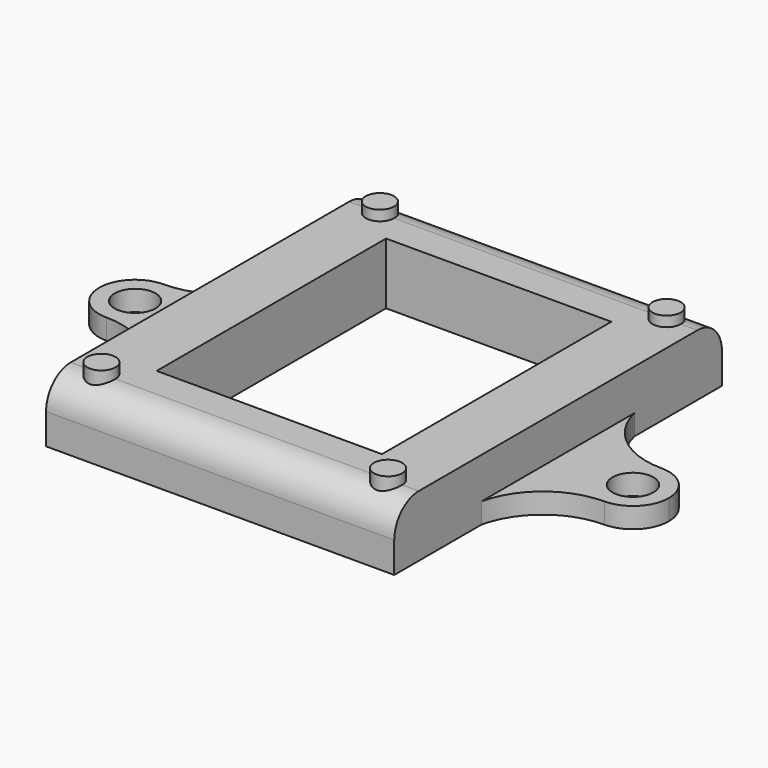
from build123d import *

# Parameters (mm, degrees)
F0_R         = 2.54
F1_DEPTH     = 2.54
F0_R_2       = 1.7526
F0_W         = 27.94
F0_H         = 35.56
F2_DEPTH     = 7.62
F3_DEPTH     = 8.89
F4_T4_DEPTH  = 62.23
F4_S5_R      = 1.7526
F4_T6_DEPTH  = 33
F4_S7_R      = 1.7526
F4_T8_DEPTH  = 33
F4_T12_DEPTH = 62.23
F4_S13_R     = 1.7526
F4_T14_DEPTH = 33
F4_S15_R     = 1.7526
F4_T16_DEPTH = 33


# Not quite as in the source:
# - a fillet or chamfer that OpenCascade refuses, or shapes differently, is made with other operations: its cross-section is extruded or revolved along the edge and cut away or added


with BuildPart() as f1:
    # F0 (on Top) → F1 (new body)
    with BuildSketch(Plane.XY):
        with BuildLine():
            ThreePointArc((-30.875, -4.445), (-24.9383449811, -6.5213926009), (-21.59, -11.8452882548))
            Line((-21.59, -11.8452882548), (-21.59, 11.8452882548))
            ThreePointArc((-21.59, 11.8452882548), (-24.9383449811, 6.5213926009), (-30.875, 4.445))
            ThreePointArc((-30.875, 4.445), (-27.7319103576, 3.1430896424), (-26.43, 0))
            ThreePointArc((-26.43, 0), (-27.7319103576, -3.1430896424), (-30.875, -4.445))
        make_face()
        with BuildLine():
            ThreePointArc((-30.875, 4.445), (-35.32, 0), (-30.875, -4.445))
            ThreePointArc((-30.875, -4.445), (-27.7319103576, -3.1430896424), (-26.43, 0))
            ThreePointArc((-26.43, 0), (-27.7319103576, 3.1430896424), (-30.875, 4.445))
        make_face()
        with Locations((-30.875, 0)):
            Circle(F0_R, mode=Mode.SUBTRACT)
    extrude(amount=F1_DEPTH)


with BuildPart() as f1b:
    # F0 (on Top) → F1, piece 2 (new body)
    with BuildSketch(Plane.XY):
        with BuildLine():
            Line((21.59, 11.8452882548), (21.59, -11.8452882548))
            ThreePointArc((21.59, -11.8452882548), (24.9383449811, -6.5213926009), (30.875, -4.445))
            ThreePointArc((30.875, -4.445), (26.43, 0), (30.875, 4.445))
            ThreePointArc((30.875, 4.445), (24.9383449811, 6.5213926009), (21.59, 11.8452882548))
        make_face()
        with BuildLine():
            ThreePointArc((30.875, 4.445), (26.43, 0), (30.875, -4.445))
            ThreePointArc((30.875, -4.445), (34.0180896424, -3.1430896424), (35.32, 0))
            ThreePointArc((35.32, 0), (34.0180896424, 3.1430896424), (30.875, 4.445))
        make_face()
        with Locations((30.875, 0)):
            Circle(F0_R, mode=Mode.SUBTRACT)
    extrude(amount=F1_DEPTH)


with BuildPart() as f2:
    # F0 (on Top) → F2 (new body)
    with BuildSketch(Plane.XY):
        Polygon((-21.59, -25.4), (21.59, -25.4), (21.59, -11.8452882548), (21.59, 11.8452882548), (21.59, 25.4), (-21.59, 25.4), (-21.59, 11.8452882548), (-21.59, -11.8452882548), align=None)
        with Locations((-17.78, -21.59)):
            Circle(F0_R_2, mode=Mode.SUBTRACT)
        with Locations((17.78, -21.59)):
            Circle(F0_R_2, mode=Mode.SUBTRACT)
        Rectangle(F0_W, F0_H, mode=Mode.SUBTRACT)
        with Locations((-17.78, 21.59)):
            Circle(F0_R_2, mode=Mode.SUBTRACT)
        with Locations((17.78, 21.59)):
            Circle(F0_R_2, mode=Mode.SUBTRACT)
    extrude(amount=F2_DEPTH)

    # F0 (on Top) → F3 (join)
    with BuildSketch(Plane.XY):
        with Locations((-17.78, 21.59)):
            Circle(F0_R_2)
        with Locations((-17.78, -21.59)):
            Circle(F0_R_2)
        with Locations((17.78, -21.59)):
            Circle(F0_R_2)
        with Locations((17.78, 21.59)):
            Circle(F0_R_2)
    extrude(amount=F3_DEPTH)

    # F4: fillet of radius 3.81 on 2 edges, made by hand


with BuildPart() as f4_tool2:
    # F4_s3 → F4_t4 (new body)
    with BuildSketch(Plane.YZ.offset(-31.115)):
        with BuildLine():
            ThreePointArc((-25.4, 3.81), (-24.2840768363, 6.5040768363), (-21.59, 7.62))
            Line((-21.59, 7.62), (-25.4, 7.62))
            Line((-25.4, 7.62), (-25.4, 3.81))
        make_face()
    extrude(amount=F4_T4_DEPTH)

    # F4_s5 → F4_t6 (cut, symmetric)
    with BuildSketch(Plane.XY.offset(5.7)):
        with Locations((-17.78, -21.59)):
            Circle(F4_S5_R)
    extrude(amount=F4_T6_DEPTH, both=True, mode=Mode.SUBTRACT)

    # F4_s7 → F4_t8 (cut, symmetric)
    with BuildSketch(Plane.XY.offset(5.7)):
        with Locations((17.78, -21.59)):
            Circle(F4_S7_R)
    extrude(amount=F4_T8_DEPTH, both=True, mode=Mode.SUBTRACT)


with BuildPart() as f2_1:
    add(f2.part)

    # F4_t1: cut F4_tool2
    add(f4_tool2.part, mode=Mode.SUBTRACT)


with BuildPart() as f4_tool10:
    # F4_s11 → F4_t12 (new body)
    with BuildSketch(Plane.YZ.offset(31.115)):
        with BuildLine():
            ThreePointArc((21.59, 7.62), (24.2840768363, 6.5040768363), (25.4, 3.81))
            Line((25.4, 3.81), (25.4, 7.62))
            Line((25.4, 7.62), (21.59, 7.62))
        make_face()
    extrude(amount=-F4_T12_DEPTH)

    # F4_s13 → F4_t14 (cut, symmetric)
    with BuildSketch(Plane.XY.offset(5.7)):
        with Locations((-17.78, 21.59)):
            Circle(F4_S13_R)
    extrude(amount=F4_T14_DEPTH, both=True, mode=Mode.SUBTRACT)

    # F4_s15 → F4_t16 (cut, symmetric)
    with BuildSketch(Plane.XY.offset(5.7)):
        with Locations((17.78, 21.59)):
            Circle(F4_S15_R)
    extrude(amount=F4_T16_DEPTH, both=True, mode=Mode.SUBTRACT)


with BuildPart() as f2_2:
    add(f2_1.part)

    # F4_t9: cut F4_tool10
    add(f4_tool10.part, mode=Mode.SUBTRACT)


solid = Compound([f1.part, f1b.part, f2_2.part])
